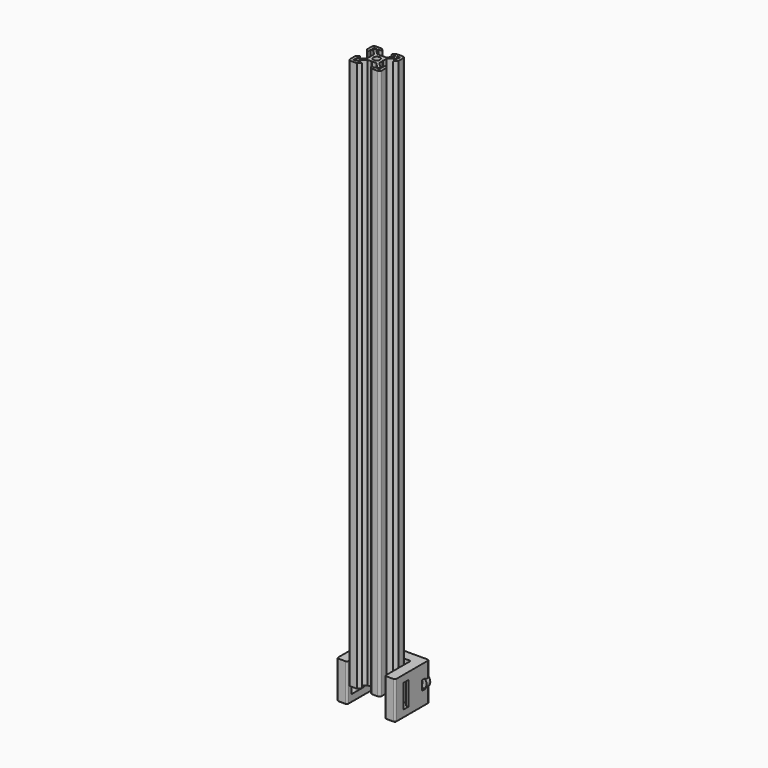
from build123d import *

# Parameters (mm, degrees)
F0_R      = 2.1
F1_DEPTH  = 310
F2_DEPTH  = 350
F8_DEPTH  = 12
F9_DEPTH  = 7.5
F10_R     = 4
F11_DEPTH = 3
F6_W      = 1.55
F6_H      = 6
F7_W      = 6.25
F7_H      = 2.6
F14_DEPTH = 3
F15_R     = 1
F16_SIZE  = 0.2


# Not quite as in the source:
# - ends of sketch curves that miss each other by under 0.0002 mm in the source are joined


with BuildPart() as f1:
    # F0 (on Top) → F1 (new body)
    with BuildSketch(Plane.XY):
        with BuildLine():
            Line((-4.64, 10.000001), (-8.500001, 10.000001))
            ThreePointArc((-8.500001, 10.000001), (-9.5606611718, 9.5606611718), (-10.000001, 8.500001))
            Line((-10.000001, 8.500001), (-10.000001, 4.64))
            Line((-10.000001, 4.64), (-8.199999, 2.84))
            Line((-8.199999, 2.84), (-8.199999, 5.499339))
            Line((-8.199999, 5.499339), (-6.56, 5.499339))
            Line((-6.56, 5.499339), (-3.90066, 2.84))
            Line((-3.90066, 2.84), (-3.90066, 0.199999))
            Line((-3.90066, 0.199999), (-3.70066, -1e-06))
            Line((-3.70066, -1e-06), (-3.90066, -0.200001))
            Line((-3.90066, -0.200001), (-3.90066, -2.840001))
            Line((-3.90066, -2.840001), (-6.56, -5.499341))
            Line((-6.56, -5.499341), (-8.199999, -5.499341))
            Line((-8.199999, -5.499341), (-8.199999, -2.840001))
            Line((-8.199999, -2.840001), (-10.000001, -4.640001))
            Line((-10.000001, -4.640001), (-10.000001, -8.500002))
            ThreePointArc((-10.000001, -8.500002), (-9.5606611718, -9.5606621718), (-8.500001, -10.000002))
            Line((-8.500001, -10.000002), (-4.64, -10.000001))
            Line((-4.64, -10.000001), (-2.84, -8.200001))
            Line((-2.84, -8.200001), (-5.49934, -8.200001))
            Line((-5.49934, -8.200001), (-5.49934, -6.560001))
            Line((-5.49934, -6.560001), (-2.84, -3.900661))
            Line((-2.84, -3.900661), (-0.199999, -3.900661))
            Line((-0.199999, -3.900661), (1e-06, -3.700661))
            Line((1e-06, -3.700661), (0.200001, -3.900661))
            Line((0.200001, -3.900661), (2.84, -3.900661))
            Line((2.84, -3.900661), (5.499342, -6.560001))
            Line((5.499342, -6.560001), (5.499342, -8.200001))
            Line((5.499342, -8.200001), (2.84, -8.200001))
            Line((2.84, -8.200001), (4.64, -10.000001))
            Line((4.64, -10.000001), (8.500001, -10.000001))
            ThreePointArc((8.500001, -10.000001), (9.5606611718, -9.5606621718), (10.000001, -8.500002))
            Line((10.000001, -8.500002), (10.000001, -4.640001))
            Line((10.000001, -4.640001), (8.200001, -2.840001))
            Line((8.200001, -2.840001), (8.200001, -5.499341))
            Line((8.200001, -5.499341), (6.560001, -5.499341))
            Line((6.560001, -5.499341), (3.90066, -2.840001))
            Line((3.90066, -2.840001), (3.90066, -0.200001))
            Line((3.90066, -0.200001), (3.70066, -1e-06))
            Line((3.70066, -1e-06), (3.90066, 0.199999))
            Line((3.90066, 0.199999), (3.90066, 2.84))
            Line((3.90066, 2.84), (6.560001, 5.499339))
            Line((6.560001, 5.499339), (8.200001, 5.499339))
            Line((8.200001, 5.499339), (8.200001, 2.84))
            Line((8.200001, 2.84), (10.000001, 4.64))
            Line((10.000001, 4.64), (10.000001, 8.500001))
            ThreePointArc((10.000001, 8.500001), (9.5606611718, 9.5606611718), (8.500001, 10.000001))
            Line((8.500001, 10.000001), (4.64, 10.000001))
            Line((4.64, 10.000001), (2.84, 8.200001))
            Line((2.84, 8.200001), (5.499342, 8.200001))
            Line((5.499342, 8.200001), (5.499342, 6.559999))
            Line((5.499342, 6.559999), (2.84, 3.90066))
            Line((2.84, 3.90066), (0.200001, 3.90066))
            Line((0.200001, 3.90066), (1e-06, 3.70066))
            Line((1e-06, 3.70066), (-0.199999, 3.90066))
            Line((-0.199999, 3.90066), (-2.84, 3.90066))
            Line((-2.84, 3.90066), (-5.49934, 6.559999))
            Line((-5.49934, 6.559999), (-5.49934, 8.200001))
            Line((-5.49934, 8.200001), (-2.84, 8.200001))
            Line((-2.84, 8.200001), (-4.64, 10.000001))
        make_face()
        Polygon((-6.56934, -8.200001), (-8.199999, -8.200001), (-8.199999, -6.569341), (-7.629999, -6.569341), (-6.56934, -7.630001), align=None, mode=Mode.SUBTRACT)
        Polygon((8.200001, -8.200001), (6.56934, -8.200001), (6.56934, -7.630001), (7.630003, -6.569341), (8.200001, -6.569341), align=None, mode=Mode.SUBTRACT)
        with Locations((1e-06, -1e-06)):
            Circle(F0_R, mode=Mode.SUBTRACT)
        Polygon((-8.199999, 8.200001), (-6.56934, 8.200001), (-6.56934, 7.63), (-7.629999, 6.56934), (-8.199999, 6.56934), align=None, mode=Mode.SUBTRACT)
        Polygon((6.56934, 8.200001), (8.200001, 8.200001), (8.200001, 6.56934), (7.630003, 6.56934), (6.56934, 7.63), align=None, mode=Mode.SUBTRACT)
    extrude(amount=F1_DEPTH)


with BuildPart() as f2:
    # F0 (on Top) → F2 (new body)
    with BuildSketch(Plane.XY):
        with BuildLine():
            Line((-4.64, 10.000001), (-8.500001, 10.000001))
            ThreePointArc((-8.500001, 10.000001), (-9.5606611718, 9.5606611718), (-10.000001, 8.500001))
            Line((-10.000001, 8.500001), (-10.000001, 4.64))
            Line((-10.000001, 4.64), (-8.199999, 2.84))
            Line((-8.199999, 2.84), (-8.199999, 5.499339))
            Line((-8.199999, 5.499339), (-6.56, 5.499339))
            Line((-6.56, 5.499339), (-3.90066, 2.84))
            Line((-3.90066, 2.84), (-3.90066, 0.199999))
            Line((-3.90066, 0.199999), (-3.70066, -1e-06))
            Line((-3.70066, -1e-06), (-3.90066, -0.200001))
            Line((-3.90066, -0.200001), (-3.90066, -2.840001))
            Line((-3.90066, -2.840001), (-6.56, -5.499341))
            Line((-6.56, -5.499341), (-8.199999, -5.499341))
            Line((-8.199999, -5.499341), (-8.199999, -2.840001))
            Line((-8.199999, -2.840001), (-10.000001, -4.640001))
            Line((-10.000001, -4.640001), (-10.000001, -8.500002))
            ThreePointArc((-10.000001, -8.500002), (-9.5606611718, -9.5606621718), (-8.500001, -10.000002))
            Line((-8.500001, -10.000002), (-4.64, -10.000001))
            Line((-4.64, -10.000001), (-2.84, -8.200001))
            Line((-2.84, -8.200001), (-5.49934, -8.200001))
            Line((-5.49934, -8.200001), (-5.49934, -6.560001))
            Line((-5.49934, -6.560001), (-2.84, -3.900661))
            Line((-2.84, -3.900661), (-0.199999, -3.900661))
            Line((-0.199999, -3.900661), (1e-06, -3.700661))
            Line((1e-06, -3.700661), (0.200001, -3.900661))
            Line((0.200001, -3.900661), (2.84, -3.900661))
            Line((2.84, -3.900661), (5.499342, -6.560001))
            Line((5.499342, -6.560001), (5.499342, -8.200001))
            Line((5.499342, -8.200001), (2.84, -8.200001))
            Line((2.84, -8.200001), (4.64, -10.000001))
            Line((4.64, -10.000001), (8.500001, -10.000001))
            ThreePointArc((8.500001, -10.000001), (9.5606611718, -9.5606621718), (10.000001, -8.500002))
            Line((10.000001, -8.500002), (10.000001, -4.640001))
            Line((10.000001, -4.640001), (8.200001, -2.840001))
            Line((8.200001, -2.840001), (8.200001, -5.499341))
            Line((8.200001, -5.499341), (6.560001, -5.499341))
            Line((6.560001, -5.499341), (3.90066, -2.840001))
            Line((3.90066, -2.840001), (3.90066, -0.200001))
            Line((3.90066, -0.200001), (3.70066, -1e-06))
            Line((3.70066, -1e-06), (3.90066, 0.199999))
            Line((3.90066, 0.199999), (3.90066, 2.84))
            Line((3.90066, 2.84), (6.560001, 5.499339))
            Line((6.560001, 5.499339), (8.200001, 5.499339))
            Line((8.200001, 5.499339), (8.200001, 2.84))
            Line((8.200001, 2.84), (10.000001, 4.64))
            Line((10.000001, 4.64), (10.000001, 8.500001))
            ThreePointArc((10.000001, 8.500001), (9.5606611718, 9.5606611718), (8.500001, 10.000001))
            Line((8.500001, 10.000001), (4.64, 10.000001))
            Line((4.64, 10.000001), (2.84, 8.200001))
            Line((2.84, 8.200001), (5.499342, 8.200001))
            Line((5.499342, 8.200001), (5.499342, 6.559999))
            Line((5.499342, 6.559999), (2.84, 3.90066))
            Line((2.84, 3.90066), (0.200001, 3.90066))
            Line((0.200001, 3.90066), (1e-06, 3.70066))
            Line((1e-06, 3.70066), (-0.199999, 3.90066))
            Line((-0.199999, 3.90066), (-2.84, 3.90066))
            Line((-2.84, 3.90066), (-5.49934, 6.559999))
            Line((-5.49934, 6.559999), (-5.49934, 8.200001))
            Line((-5.49934, 8.200001), (-2.84, 8.200001))
            Line((-2.84, 8.200001), (-4.64, 10.000001))
        make_face()
        Polygon((-6.56934, -8.200001), (-8.199999, -8.200001), (-8.199999, -6.569341), (-7.629999, -6.569341), (-6.56934, -7.630001), align=None, mode=Mode.SUBTRACT)
        Polygon((8.200001, -8.200001), (6.56934, -8.200001), (6.56934, -7.630001), (7.630003, -6.569341), (8.200001, -6.569341), align=None, mode=Mode.SUBTRACT)
        with Locations((1e-06, -1e-06)):
            Circle(F0_R, mode=Mode.SUBTRACT)
        Polygon((-8.199999, 8.200001), (-6.56934, 8.200001), (-6.56934, 7.63), (-7.629999, 6.56934), (-8.199999, 6.56934), align=None, mode=Mode.SUBTRACT)
        Polygon((6.56934, 8.200001), (8.200001, 8.200001), (8.200001, 6.56934), (7.630003, 6.56934), (6.56934, 7.63), align=None, mode=Mode.SUBTRACT)
    extrude(amount=F2_DEPTH)


with BuildPart() as f8:
    # F4 (on Top) → F8 (new body, symmetric)
    with BuildSketch(Plane.XY):
        Polygon((18.500001, 18.500001), (-18.500001, 18.500001), (-18.500001, -8.500002), (-12.000001, -8.500002), (-12.000001, 12.000001), (12.000001, 12.000001), (12.000001, -8.500002), (18.500001, -8.500002), align=None)
    extrude(amount=F8_DEPTH, both=True)

    # F5 (on Top) → F9 (cut, symmetric)
    with BuildSketch(Plane.XY):
        with BuildLine():
            ThreePointArc((-17.0773353328, -2), (-15.2832682204, -4.0846607111), (-12.645190677, -4.8625))
            Line((-12.645190677, -4.8625), (-4.8625, -4.8625))
            Line((-4.8625, -4.8625), (-4.8625, -10.4973195121))
            ThreePointArc((-4.8625, -10.4973195121), (0, -15.3598195121), (4.8625, -10.4973195121))
            Line((4.8625, -10.4973195121), (4.8625, -4.8625))
            Line((4.8625, -4.8625), (12.645190677, -4.8625))
            ThreePointArc((12.645190677, -4.8625), (15.2832682204, -4.0846607111), (17.0773353328, -2))
            ThreePointArc((17.0773353328, -2), (17.507690677, 0), (17.0773353328, 2))
            ThreePointArc((17.0773353328, 2), (15.2832682204, 4.0846607111), (12.645190677, 4.8625))
            Line((12.645190677, 4.8625), (4.8625, 4.8625))
            Line((4.8625, 4.8625), (4.8625, 12.6451930908))
            ThreePointArc((4.8625, 12.6451930908), (4.0846607111, 15.2832706342), (2, 17.0773377466))
            ThreePointArc((2, 17.0773377466), (0, 17.5076930908), (-2, 17.0773377466))
            ThreePointArc((-2, 17.0773377466), (-4.0846607111, 15.2832706342), (-4.8625, 12.6451930908))
            Line((-4.8625, 12.6451930908), (-4.8625, 4.8625))
            Line((-4.8625, 4.8625), (-12.645190677, 4.8625))
            ThreePointArc((-12.645190677, 4.8625), (-15.2832682204, 4.0846607111), (-17.0773353328, 2))
            ThreePointArc((-17.0773353328, 2), (-17.507690677, 0), (-17.0773353328, -2))
        make_face()
        with BuildLine():
            Line((-24.7247423977, -2), (-17.0773353328, -2))
            ThreePointArc((-17.0773353328, -2), (-17.507690677, 0), (-17.0773353328, 2))
            Line((-17.0773353328, 2), (-24.7247423977, 2))
            Line((-24.7247423977, 2), (-24.7247423977, -2))
        make_face()
        with BuildLine():
            Line((-2, 25.2566821873), (-2, 17.0773377466))
            ThreePointArc((-2, 17.0773377466), (0, 17.5076930908), (2, 17.0773377466))
            Line((2, 17.0773377466), (2, 25.2566821873))
            Line((2, 25.2566821873), (-2, 25.2566821873))
        make_face()
        with BuildLine():
            ThreePointArc((17.0773353328, 2), (17.507690677, 0), (17.0773353328, -2))
            Line((17.0773353328, -2), (24.7247423977, -2))
            Line((24.7247423977, -2), (24.7247423977, 2))
            Line((24.7247423977, 2), (17.0773353328, 2))
        make_face()
    extrude(amount=F9_DEPTH, both=True, mode=Mode.SUBTRACT)

    # F10 (on face) → F11 (join)
    with BuildSketch(Plane(origin=(0, 18.500001, 0), x_dir=(-1, 0, 0), z_dir=(0, 1, 0))):
        with Locations((-15.250001, 0)):
            Circle(F10_R)
        with Locations((15.250001, 0)):
            Circle(F10_R)
    extrude(amount=-F11_DEPTH)

    # F6 (on Top) → F12 (revolve, cut)
    with BuildSketch(Plane.XY):
        with Locations((-16.025001, 15.500001)):
            Rectangle(F6_W, F6_H)
    revolve(axis=Axis((-15.250001, 15.500001, 0), (0, -1, 0)), mode=Mode.SUBTRACT)

    # F6 (on Top) → F13 (revolve, cut)
    with BuildSketch(Plane.XY):
        with Locations((16.025001, 15.500001)):
            Rectangle(F6_W, F6_H)
    revolve(axis=Axis((15.250001, 15.500001, 0), (0, -1, 0)), mode=Mode.SUBTRACT)

    # F7 (on Top) → F14 (cut, symmetric)
    with BuildSketch(Plane.XY):
        with Locations((-15.375001, 14.200001)):
            Rectangle(F7_W, F7_H)
        with Locations((15.375001, 14.200001)):
            Rectangle(F7_W, F7_H)
    extrude(amount=F14_DEPTH, both=True, mode=Mode.SUBTRACT)

    # F15
    f15_edges = [f8.edges().sort_by_distance(p)[0] for p in [
        (-18.500001, 18.500001, -7.165922),
        (-18.500001, 18.500001, 7.165922),
        (-18.500001, -8.500002, 0),
        (-12.000001, -8.500002, 0),
        (12.000001, -8.500002, 0),
        (18.500001, -8.500002, 0),
        (12.000001, 12.000001, 0),
        (-12.000001, 12.000001, 0),
        (18.500001, 18.500001, -7.165922),
        (18.500001, 18.500001, 7.165922),
    ]]
    fillet(f15_edges, radius=F15_R)

    # F16
    f16_edges = [f8.edges().sort_by_distance(p)[0] for p in [
        (0, 18.500001, -12),
        (18.207108, 18.207108, -12),
        (-18.207108, 18.207108, -12),
        (18.500001, 4.999999, -12),
        (-18.500001, 5, -12),
        (18.207108, -8.207109, -12),
        (-18.207108, -8.207109, -12),
        (15.250001, -8.500002, -12),
        (-15.250001, -8.500002, -12),
        (12.292894, -8.207109, -12),
        (-12.292894, -8.207109, -12),
        (12.000001, 1.749999, -12),
        (-12.000001, 1.749999, -12),
        (11.707108, 11.707108, -12),
        (-11.707108, 11.707108, -12),
        (0, 12.000001, -12),
    ]]
    chamfer(f16_edges, length=F16_SIZE)


solid = Compound([f1.part, f2.part, f8.part])
